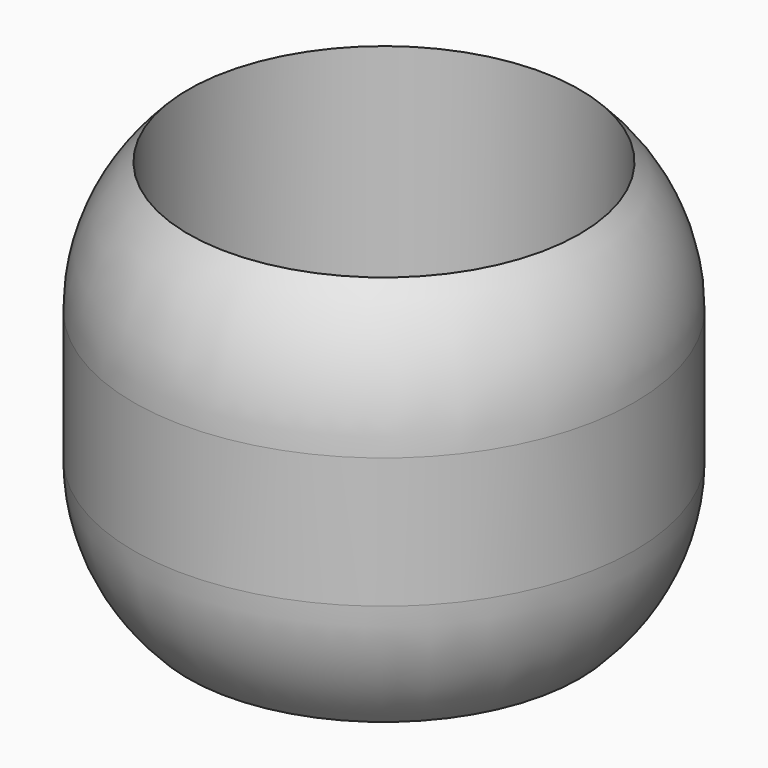
from build123d import *

# Parameters (mm, degrees)
F0_R     = 97.536
F0_R_2   = 76.2
F1_DEPTH = 152.4


# Not quite as in the source:
# - a fillet or chamfer that OpenCascade refuses, or shapes differently, is made with other operations: its cross-section is extruded or revolved along the edge and cut away or added


with BuildPart() as f1:
    # F0 (on Top) → F1 (new body)
    with BuildSketch(Plane.XY):
        Circle(F0_R)
        Circle(F0_R_2, mode=Mode.SUBTRACT)
    extrude(amount=F1_DEPTH)

    # F2: fillet of radius 71.12 on 1 edges, made by hand

    # F2_s1 → F2_t2 (revolve, cut)
    with BuildSketch(Plane.XZ):
        with BuildLine():
            ThreePointArc((97.536, 101.6101610162), (91.9854001803, 129.1548185744), (76.2, 152.4))
            Line((76.2, 152.4), (97.536, 152.4))
            Line((97.536, 152.4), (97.536, 101.6101610162))
        make_face()
    revolve(axis=Axis((0, 0, 152.4), (0, 0, 1)), mode=Mode.SUBTRACT)

    # F3: fillet of radius 71.12 on 3 edges, made by hand

    # F3_s1 → F3_t2 (revolve, cut)
    with BuildSketch(Plane.XZ):
        with BuildLine():
            ThreePointArc((97.536, 50.7898389838), (91.9854001803, 23.2451814256), (76.2, 0))
            Line((76.2, 0), (97.536, 0))
            Line((97.536, 0), (97.536, 50.7898389838))
        make_face()
    revolve(axis=Axis((0, 0, 0), (0, 0, 1)), mode=Mode.SUBTRACT)


solid = f1.part
